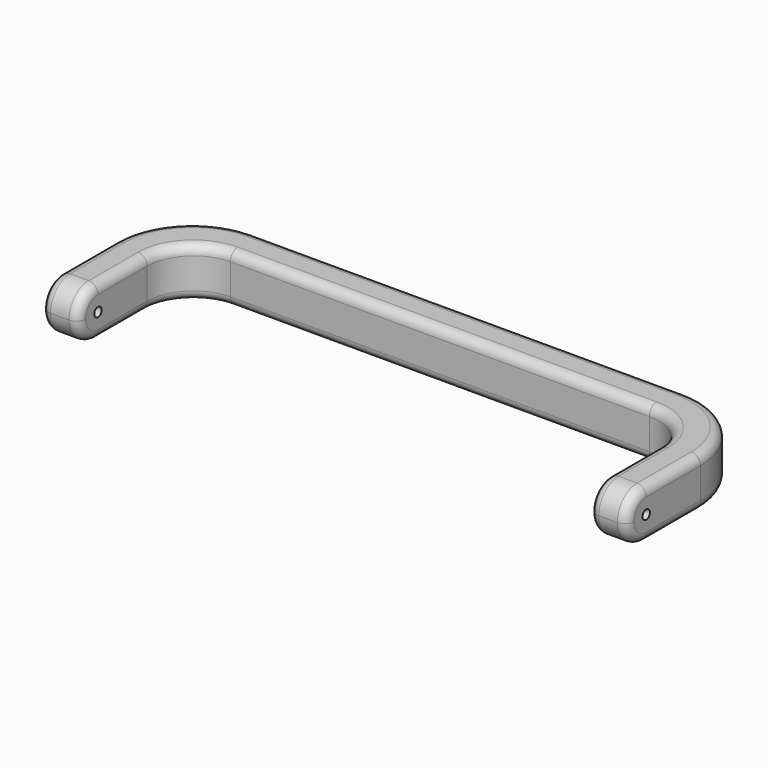
from build123d import *

# Parameters (mm, degrees)
F1_DEPTH = 16
F2_R     = 15
F3_R     = 25
F4_R     = 7.99999
F5_R     = 1.5
F6_DEPTH = 250
F7_R     = 3


# Not quite as in the source:
# - a fillet or chamfer is up to 0.001 mm smaller than in the source, because OpenCascade refuses the exact size


with BuildPart() as f1:
    # F0 (on Top) → F1 (new body)
    with BuildSketch(Plane.XY):
        Polygon((95, 35.7796452148), (0, 35.7796452148), (-95, 35.7796452148), (-95, -19.2203547852), (-83, -19.2203547852), (-83, 23.7796452148), (0, 23.7796452148), (83, 23.7796452148), (83, -19.2203547852), (95, -19.2203547852), align=None)
    extrude(amount=F1_DEPTH)

    # F2
    f2_edges = [f1.edges().sort_by_distance(p)[0] for p in [
        (-83, 23.779645, 8),
        (83, 23.779645, 8),
    ]]
    fillet(f2_edges, radius=F2_R)

    # F3
    f3_edges = [f1.edges().sort_by_distance(p)[0] for p in [
        (-95, 35.779645, 8),
        (95, 35.779645, 8),
    ]]
    fillet(f3_edges, radius=F3_R)

    # F4 (radius 8 in the source; OpenCascade refuses exactly that, so slightly less here)
    f4_edges = [f1.edges().sort_by_distance(p)[0] for p in [
        (-89, -19.220355, 16),
        (-89, -19.220355, 0),
        (89, -19.220355, 16),
        (89, -19.220355, 0),
    ]]
    fillet(f4_edges, radius=F4_R)

    # F5 (on face) → F6 (cut)
    with BuildSketch(Plane.YZ.offset(95)):
        with Locations((-11.2203547852, 8)):
            Circle(F5_R)
    extrude(amount=-F6_DEPTH, mode=Mode.SUBTRACT)

    # F7
    f7_edges = [f1.edges().sort_by_distance(p)[0] for p in [
        (-95, -0.22036, 0),
        (-89, -11.220365, 0),
        (-87.67767, 28.457315, 0),
        (-83, -1.22036, 0),
        (0, 35.779645, 0),
        (-78.606602, 19.386247, 0),
        (87.67767, 28.457315, 0),
        (0, 23.779645, 0),
        (95, -0.22036, 0),
        (78.606602, 19.386247, 0),
        (89, -11.220365, 0),
        (83, -1.22036, 0),
    ]]
    fillet(f7_edges, radius=F7_R)


solid = f1.part
